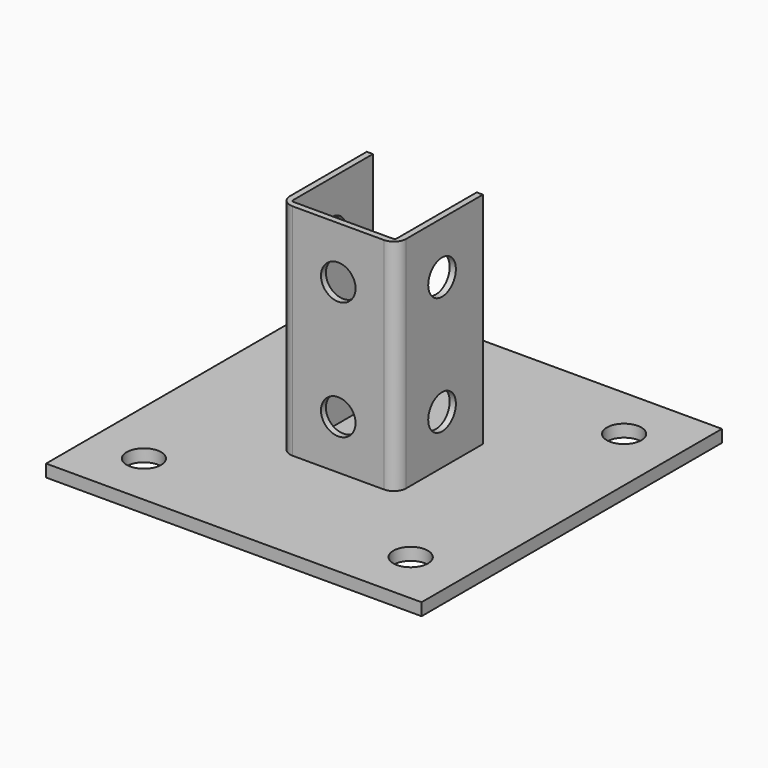
from build123d import *

# Parameters (mm, degrees)
F0_W     = 152
F0_H     = 152
F0_R     = 7
F1_DEPTH = 5
F3_DEPTH = 88.9
F4_R     = 5
F5_R     = 1
F7_D     = 14
F9_D     = 14


# Not quite as in the source:
# - a feature names something its author has since deleted; it is built from what else it names


with BuildPart() as f1:
    # F0 (on Top) → F1 (new body)
    with BuildSketch(Plane.XY):
        Rectangle(F0_W, F0_H)
        with Locations((-54, -54)):
            Circle(F0_R, mode=Mode.SUBTRACT)
        with Locations((54, -54)):
            Circle(F0_R, mode=Mode.SUBTRACT)
        with Locations((-54, 54)):
            Circle(F0_R, mode=Mode.SUBTRACT)
        with Locations((54, 54)):
            Circle(F0_R, mode=Mode.SUBTRACT)
    extrude(amount=-F1_DEPTH)

    # F2 (on face) → F3 (join)
    with BuildSketch(Plane.XY):
        Polygon((-21, 20.65), (-23.5, 20.65), (-23.5, -23.15), (23.5, -23.15), (23.5, 20.65), (21, 20.65), (21, -20.65), (-21, -20.65), align=None)
    extrude(amount=F3_DEPTH)

    # F4
    f4_edges = [f1.edges().sort_by_distance(p)[0] for p in [
        (23.5, -23.15, 44.45),
        (-23.5, -23.15, 44.45),
    ]]
    fillet(f4_edges, radius=F4_R)

    # F5
    f5_edges = [f1.edges().sort_by_distance(p)[0] for p in [
        (21, -20.65, 44.45),
        (-21, -20.65, 44.45),
    ]]
    fillet(f5_edges, radius=F5_R)

    # F7 (through all)
    with Locations(Plane.YZ.offset(23.5)):
        with Locations((0, 67.9), (0, 19.9)):
            Hole(F7_D / 2)

    # F9 (through all)
    with Locations(Plane.XZ.offset(23.15)):
        with Locations((0, 67.9), (0, 19.9)):
            Hole(F9_D / 2)


solid = f1.part
